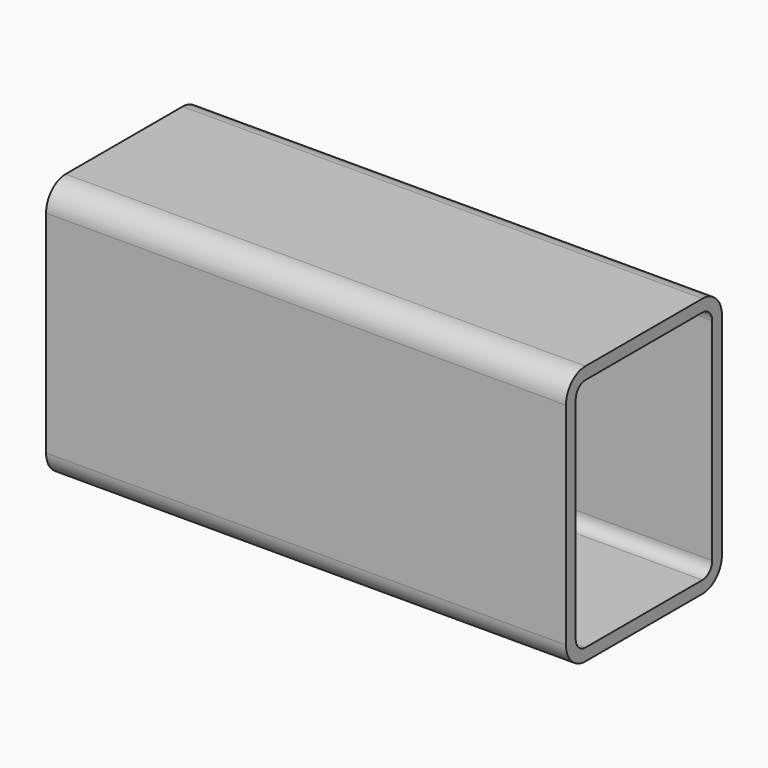
from build123d import *

# Parameters (mm, degrees)
F2_DEPTH = 101.6


# Not quite as in the source:
# - a variable given as a bare number and used for a length is read in inches; the dataset says mm whatever the document's units were


with BuildPart() as f2:
    # F1 (on Right) → F2 (new body, symmetric)
    with BuildSketch(Plane.YZ):
        with BuildLine():
            Line((28.575, 50.8), (-28.575, 50.8))
            ThreePointArc((-28.575, 50.8), (-35.3101920908, 48.0101920908), (-38.1, 41.275))
            Line((-38.1, 41.275), (-38.1, -41.275))
            ThreePointArc((-38.1, -41.275), (-35.3101920908, -48.0101920908), (-28.575, -50.8))
            Line((-28.575, -50.8), (28.575, -50.8))
            ThreePointArc((28.575, -50.8), (35.3101920908, -48.0101920908), (38.1, -41.275))
            Line((38.1, -41.275), (38.1, 41.275))
            ThreePointArc((38.1, 41.275), (35.3101920908, 48.0101920908), (28.575, 50.8))
        make_face()
        with BuildLine():
            ThreePointArc((-33.3375, 41.275), (-31.9425960454, 44.6425960454), (-28.575, 46.0375))
            Line((-28.575, 46.0375), (28.575, 46.0375))
            ThreePointArc((28.575, 46.0375), (31.9425960454, 44.6425960454), (33.3375, 41.275))
            Line((33.3375, 41.275), (33.3375, -41.275))
            ThreePointArc((33.3375, -41.275), (31.9425960454, -44.6425960454), (28.575, -46.0375))
            Line((28.575, -46.0375), (-28.575, -46.0375))
            ThreePointArc((-28.575, -46.0375), (-31.9425960454, -44.6425960454), (-33.3375, -41.275))
            Line((-33.3375, -41.275), (-33.3375, 41.275))
        make_face(mode=Mode.SUBTRACT)
    extrude(amount=F2_DEPTH, both=True)


solid = f2.part
